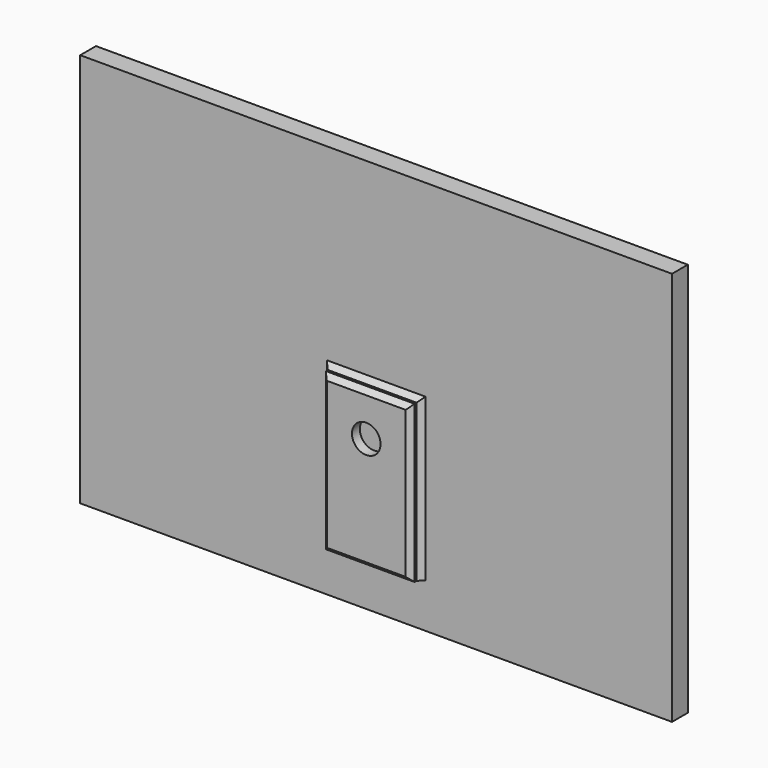
from build123d import *

# Parameters (mm, degrees)
F0_W         = 600
F0_H         = 400
F0_W_2       = 550
F0_H_2       = 330
F1_DEPTH     = 20
F2_W         = 90
F2_H         = 159.0613481622
F3_DEPTH     = 12.5
F4_DEPTH     = 15
F5_SIZE      = 5
F6_R         = 14.5
F7_DEPTH     = 10
F8_TEXT_SIZE = 177.5050018397
F9_DEPTH     = 10


# Not quite as in the source:
# - Text() gives the source's letters only with a copy of the font that has no kerning and outlines rounded to 1/6400 em; it was checked with that copy


with BuildPart() as f1:
    # F0 (on Front) → F1 (new body)
    with BuildSketch(Plane.XZ):
        with Locations((0, 155)):
            Rectangle(F0_W, F0_H)
        with Locations((0, 165)):
            Rectangle(F0_W_2, F0_H_2, mode=Mode.SUBTRACT)
    extrude(amount=-F1_DEPTH)

    # F2 (on face) → F3 (join, symmetric)
    with BuildSketch(Plane.XZ):
        with Locations((0, 79.5306740811)):
            Rectangle(F2_W, F2_H)
    extrude(amount=F3_DEPTH, both=True)

    # F0 (on Front) → F4 (join)
    with BuildSketch(Plane.XZ):
        with Locations((0, 165)):
            Rectangle(F0_W_2, F0_H_2)
    extrude(amount=-F4_DEPTH)

    # F5
    f5_edges = [f1.edges().sort_by_distance(p)[0] for p in [
        (0, -12.5, 159.061348),
        (-45, -12.5, 79.530674),
        (0, -12.5, 0),
        (45, -12.5, 79.530674),
        (45, 0, 79.530674),
        (-45, 0, 79.530674),
        (0, 0, 159.061348),
    ]]
    chamfer(f5_edges, length=F5_SIZE)

    # F6 (on face) → F7 (cut)
    with BuildSketch(Plane.XZ.offset(12.5)):
        with Locations((0, 115.1828020811)):
            Circle(F6_R)
    extrude(amount=-F7_DEPTH, mode=Mode.SUBTRACT)

    # F8 (on face) → F9 (join)
    with BuildSketch(Plane(origin=(0, 15, 0), x_dir=(-1, 0, 0), z_dir=(0, 1, 0))):
        with Locations((-190.7707825303, 119.3455085158)):
            Text('E J H', F8_TEXT_SIZE, font='Open Sans', font_style=FontStyle.BOLDITALIC, text_align=(TextAlign.LEFT, TextAlign.BOTTOM))
    extrude(amount=F9_DEPTH)


solid = f1.part
